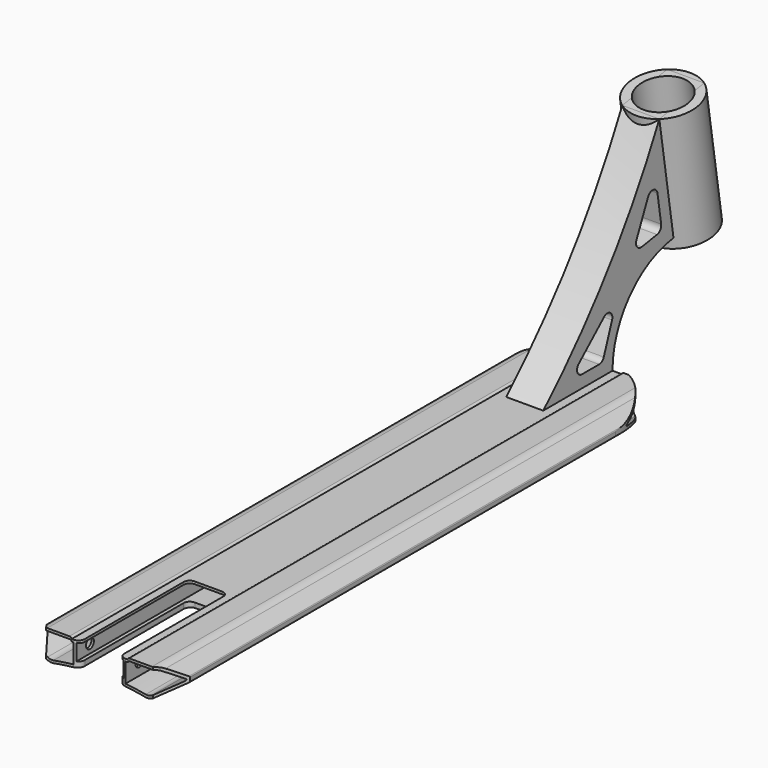
from build123d import *

# Parameters (mm, degrees)
F1_DEPTH       = 250
F2_W           = 38
F2_H           = 13
F3_DEPTH       = 250
F4_T1_DEPTH    = 509.3674969976
F5_R           = 9
F6_R           = 1
F8_DEPTH       = 500.001
F10_DEPTH      = 1.301
F10_DEPTH_BACK = 22.2193051812
F12_DEPTH      = 22.219305294
F12_DEPTH_BACK = 1.3010001
F13_T1_DEPTH   = 2
F13_T6_DEPTH   = 16.7634824315
F13_S7_R       = 200
F13_T8_DEPTH   = 11
F13_T12_DEPTH  = 16.7634824315
F13_S13_R      = 200
F13_T14_DEPTH  = 11
F13_T15_DEPTH  = 27
F13_T17_DEPTH  = 29.2634824315
F15_DEPTH      = 15
F16_R          = 27.4590604355
F17_DEPTH      = 100
F19_D          = 40
F21_D          = 8
F21_DEPTH      = 50
F21_TIP        = 2.4034424761
F23_DEPTH      = 72.5010001
F24_R          = 5


# Not quite as in the source:
# - a fillet or chamfer that OpenCascade refuses, or shapes differently, is made with other operations: its cross-section is extruded or revolved along the edge and cut away or added


with BuildPart() as f1:
    # F0 (on Front) → F1 (new body, symmetric)
    with BuildSketch(Plane.XZ):
        with BuildLine():
            Line((22.5, 0), (0, 0))
            Line((0, 0), (-22.5, 0))
            Line((-22.5, 0), (-22.5, 1.3))
            Line((-22.5, 1.3), (-45.5824640741, 1.3))
            Line((-45.5824640741, 1.3), (-57.5, -8.7))
            Line((-57.5, -8.7), (-57.5, -12.7))
            Line((-57.5, -12.7), (-40.1794919243, -22.7))
            ThreePointArc((-40.1794919243, -22.7), (0, -18.6224551416), (40.1794919243, -22.7))
            Line((40.1794919243, -22.7), (57.5, -12.7))
            Line((57.5, -12.7), (57.5, -8.7))
            Line((57.5, -8.7), (45.5824640741, 1.3))
            Line((45.5824640741, 1.3), (22.5, 1.3))
            Line((22.5, 1.3), (22.5, 0))
        make_face()
    extrude(amount=F1_DEPTH, both=True)

    # F2 (on Front) → F3 (cut, symmetric)
    with BuildSketch(Plane.XZ):
        with Locations((0, -8.5)):
            Rectangle(F2_W, F2_H)
    extrude(amount=F3_DEPTH, both=True, mode=Mode.SUBTRACT)

    # F4: fillet of radius 2 on 2 edges, made by hand

    # F4_s2 → F4_t1 (cut)
    with BuildSketch(Plane.XZ.offset(-254.6837484988)):
        with BuildLine():
            ThreePointArc((24.3734993995, 1.3), (23.2333239744, 0.9431676725), (22.5, 0))
            Line((22.5, 0), (22.5, 1.3))
            Line((22.5, 1.3), (24.3734993995, 1.3))
        make_face()
        with BuildLine():
            ThreePointArc((-24.3734993995, 1.3), (-23.2333239744, 0.9431676725), (-22.5, 0))
            Line((-22.5, 0), (-22.5, 1.3))
            Line((-22.5, 1.3), (-24.3734993995, 1.3))
        make_face()
    extrude(amount=F4_T1_DEPTH, mode=Mode.SUBTRACT)

    # F5
    f5_edges = [f1.edges().sort_by_distance(p)[0] for p in [
        (45.582464, 0, 1.3),
        (-45.582464, 0, 1.3),
        (40.179492, 0, -22.7),
        (-40.179492, 0, -22.7),
    ]]
    fillet(f5_edges, radius=F5_R)

    # F6
    f6_edges = [f1.edges().sort_by_distance(p)[0] for p in [
        (57.5, 0, -8.7),
        (57.5, 0, -12.7),
        (-57.5, 0, -8.7),
        (-57.5, 0, -12.7),
    ]]
    fillet(f6_edges, radius=F6_R)

    # F7 (on face) → F8 (cut, through all)
    with BuildSketch(Plane.XZ.offset(250)):
        with BuildLine():
            ThreePointArc((-37.3093701274, -20.0978700124), (-29.1789785809, -18.7410222645), (-21, -17.7170047426))
            Line((-21, -17.7170047426), (-21, -2))
            Line((-21, -2), (-22.5, -2))
            ThreePointArc((-22.5, -2), (-23.2333239744, -1.0568323275), (-24.3734993995, -0.7))
            Line((-24.3734993995, -0.7), (-42.3067319657, -0.7))
            ThreePointArc((-42.3067319657, -0.7), (-44.7008729689, -1.1221516545), (-46.8062452335, -2.3376888982))
            Line((-46.8062452335, -2.3376888982), (-55.7563117574, -9.8476864174))
            ThreePointArc((-55.7563117574, -9.8476864174), (-56.1097188459, -10.7008866033), (-55.6135241478, -11.4797562644))
            Line((-55.6135241478, -11.4797562644), (-42.1022690923, -19.2804830077))
            ThreePointArc((-42.1022690923, -19.2804830077), (-39.7790673433, -20.1186780608), (-37.3093701274, -20.0978700124))
        make_face()
        with BuildLine():
            ThreePointArc((21, -17.7170047426), (29.1789785809, -18.7410222645), (37.3093701274, -20.0978700124))
            ThreePointArc((37.3093701274, -20.0978700124), (39.7790673433, -20.1186780608), (42.1022690923, -19.2804830077))
            Line((42.1022690923, -19.2804830077), (55.6135241478, -11.4797562644))
            ThreePointArc((55.6135241478, -11.4797562644), (56.1097188459, -10.7008866033), (55.7563117574, -9.8476864174))
            Line((55.7563117574, -9.8476864174), (46.8062452335, -2.3376888982))
            ThreePointArc((46.8062452335, -2.3376888982), (44.7008729689, -1.1221516545), (42.3067319657, -0.7))
            Line((42.3067319657, -0.7), (24.3734993995, -0.7))
            ThreePointArc((24.3734993995, -0.7), (23.2333239744, -1.0568323275), (22.5, -2))
            Line((22.5, -2), (21, -2))
            Line((21, -2), (21, -17.7170047426))
        make_face()
    extrude(amount=-F8_DEPTH, mode=Mode.SUBTRACT)

    # F9 (on Top) → F10 (cut, two sides)
    with BuildSketch(Plane.XY) as f10_sk:
        with BuildLine():
            ThreePointArc((-57.5, 200), (0, 257.5), (57.5, 200))
            Line((57.5, 200), (57.5, 280))
            Line((57.5, 280), (-57.5, 280))
            Line((-57.5, 280), (-57.5, 200))
        make_face()
    extrude(amount=F10_DEPTH, mode=Mode.SUBTRACT)
    extrude(f10_sk.sketch, amount=-F10_DEPTH_BACK, mode=Mode.SUBTRACT)

    # F11 (on Top) → F12 (cut, two sides)
    with BuildSketch(Plane.XY) as f12_sk:
        Polygon((-43.2975540478, -250), (-68, -216), (-68, -346), (68, -346), (68, -216), (43.2975540478, -250), (16, -250), (16, -140), (-16, -140), (-16, -250), align=None)
    extrude(amount=-F12_DEPTH, mode=Mode.SUBTRACT)
    extrude(f12_sk.sketch, amount=F12_DEPTH_BACK, mode=Mode.SUBTRACT)

    # F13: fillet of radius 5 on 8 edges, made by hand

    # F13_s2 → F13_t1 (join)
    with BuildSketch(Plane.XY.offset(-2)):
        with BuildLine():
            ThreePointArc((-11, -140), (-14.5355339059, -141.4644660941), (-16, -145))
            Line((-16, -145), (-16, -140))
            Line((-16, -140), (-11, -140))
        make_face()
        with BuildLine():
            ThreePointArc((16, -145), (14.5355339059, -141.4644660941), (11, -140))
            Line((11, -140), (16, -140))
            Line((16, -140), (16, -145))
        make_face()
    extrude(amount=F13_T1_DEPTH)


with BuildPart() as f13_tool4:
    # F13_s5 → F13_t6 (new body)
    with BuildSketch(Plane.XY.offset(-15)):
        with BuildLine():
            ThreePointArc((-16, -145), (-14.5355339059, -141.4644660941), (-11, -140))
            Line((-11, -140), (-16, -140))
            Line((-16, -140), (-16, -145))
        make_face()
    extrude(amount=-F13_T6_DEPTH)

    # F13_s7 → F13_t8 (cut, symmetric)
    with BuildSketch(Plane.XZ.offset(142.5)):
        with Locations((0, -218.6224551416)):
            Circle(F13_S7_R)
    extrude(amount=F13_T8_DEPTH, both=True, mode=Mode.SUBTRACT)


with BuildPart() as f1_1:
    add(f1.part)

    # F13_t3: union F13_tool4
    add(f13_tool4.part)


with BuildPart() as f13_tool10:
    # F13_s11 → F13_t12 (new body)
    with BuildSketch(Plane.XY.offset(-31.7634824315)):
        with BuildLine():
            ThreePointArc((11, -140), (14.5355339059, -141.4644660941), (16, -145))
            Line((16, -145), (16, -140))
            Line((16, -140), (11, -140))
        make_face()
    extrude(amount=F13_T12_DEPTH)

    # F13_s13 → F13_t14 (cut, symmetric)
    with BuildSketch(Plane.XZ.offset(142.5)):
        with Locations((0, -218.6224551416)):
            Circle(F13_S13_R)
    extrude(amount=F13_T14_DEPTH, both=True, mode=Mode.SUBTRACT)


with BuildPart() as f1_2:
    add(f1_1.part)

    # F13_t9: union F13_tool10
    add(f13_tool10.part)

    # F13_s16 → F13_t15 (cut)
    with BuildSketch(Plane.XY.offset(-14.5)):
        with BuildLine():
            ThreePointArc((-21, -250), (-17.4644660941, -248.5355339059), (-16, -245))
            Line((-16, -245), (-16, -250))
            Line((-16, -250), (-21, -250))
        make_face()
        with BuildLine():
            ThreePointArc((21, -250), (17.4644660941, -248.5355339059), (16, -245))
            Line((16, -245), (16, -250))
            Line((16, -250), (21, -250))
        make_face()
    extrude(amount=F13_T15_DEPTH, mode=Mode.SUBTRACT)

    # F13_s18 → F13_t17 (cut)
    with BuildSketch(Plane.XY.offset(-31.7634824315)):
        with BuildLine():
            ThreePointArc((-21, -250), (-17.4644660941, -248.5355339059), (-16, -245))
            Line((-16, -245), (-16, -250))
            Line((-16, -250), (-21, -250))
        make_face()
        with BuildLine():
            ThreePointArc((21, -250), (17.4644660941, -248.5355339059), (16, -245))
            Line((16, -245), (16, -250))
            Line((16, -250), (21, -250))
        make_face()
    extrude(amount=F13_T17_DEPTH, mode=Mode.SUBTRACT)

    # F14 (on Right) → F15 (join, symmetric)
    with BuildSketch(Plane.YZ):
        with BuildLine():
            Line((180, 0), (250, 0))
            ThreePointArc((250, 0), (267.6550746197, 46.4758946867), (311.7145367693, 69.5079211245))
            Line((311.7145367693, 69.5079211245), (313.0254460068, 61.2311659405))
            Line((313.0254460068, 61.2311659405), (358.4591096742, 68.4271513323))
            Line((358.4591096742, 68.4271513323), (342.8156631702, 167.1959853919))
            Line((342.8156631702, 167.1959853919), (297.3819995028, 160))
            ThreePointArc((297.3819995028, 160), (245.9666940414, 74.662277853), (180, 0))
        make_face()
    extrude(amount=F15_DEPTH, both=True)

    # F16 (on face) → F17 (join, through all)
    with BuildSketch(Plane(origin=(0, -17.4439040266, 110.1364754698), x_dir=(1, 0, 0), z_dir=(0, -0.156434465, 0.9876883406))):
        with Locations((0, 341.7502480182)):
            Circle(F16_R)
    extrude(amount=-F17_DEPTH)

    # F19 (through all)
    with Locations(Plane(origin=(0, -17.4439040266, 110.1364754698), x_dir=(1, 0, 0), z_dir=(0, -0.156434465, 0.9876883406))):
        with Locations((0, 341.7502480182)):
            Hole(F19_D / 2)

    # F21 (one way)
    with BuildSketch(Plane.YZ.offset(21)):
        with Locations((-236, -7.7170047426)):
            Circle(F21_D / 2)
    extrude(amount=-F21_DEPTH, mode=Mode.SUBTRACT)
    with Locations(Plane.YZ.offset(21)):
        with Locations((-236, -7.7170047426)):
            with Locations((0, 0, -(F21_DEPTH + F21_TIP / 2))):  # 118° drill point
                Cone(0, F21_D / 2, F21_TIP, mode=Mode.SUBTRACT)

    # F22 (on face) → F23 (cut, through all)
    with BuildSketch(Plane.YZ.offset(15)):
        Polygon((256.378660542, 55), (206, 10), (240, 10), align=None)
        Polygon((292.8925734855, 124.4205881019), (270.3892230822, 74.7275541507), (300.0198733001, 79.4205881019), align=None)
    extrude(amount=-F23_DEPTH, mode=Mode.SUBTRACT)

    # F24
    f24_edges = [f1_2.edges().sort_by_distance(p)[0] for p in [
        (0, 292.892573, 124.420588),
        (0, 270.389223, 74.727554),
        (0, 300.019873, 79.420588),
        (0, 240, 10),
        (0, 206, 10),
        (0, 256.378661, 55),
    ]]
    fillet(f24_edges, radius=F24_R)


solid = f1_2.part
